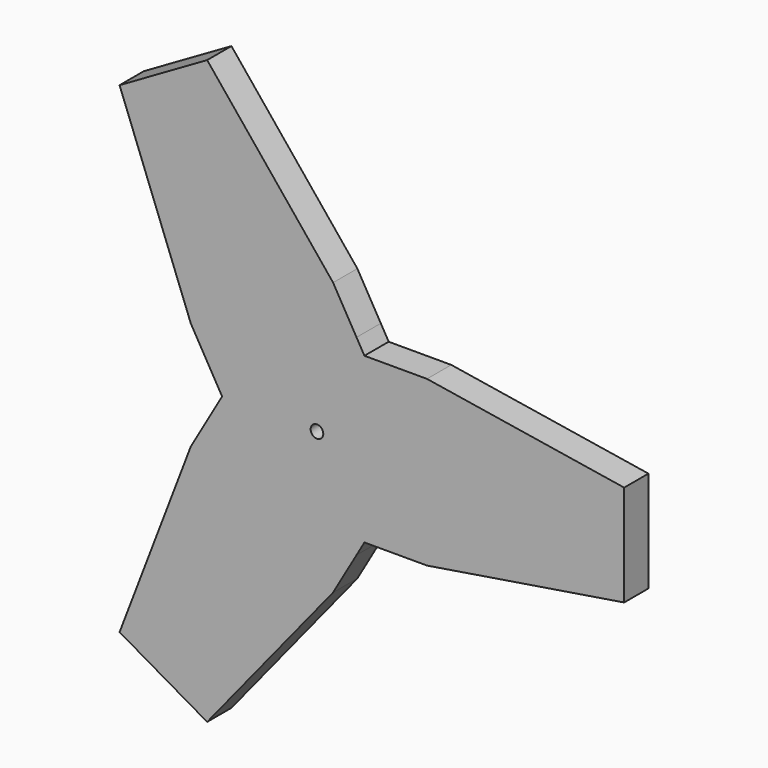
from build123d import *

# Parameters (mm, degrees)
F1_DEPTH = 6
F2_R     = 2.5
F3_DEPTH = 12.001


# Not quite as in the source:
# - a feature names something its author has since deleted; it is built from what else it names


with BuildPart() as f1:
    # F0 (on Front) → F1 (new body, symmetric)
    with BuildSketch(Plane.XZ):
        Polygon((43.524, -32.5), (121.5, -20), (121.5, 20), (43.524, 32.5), (25, 32.5), (18.7638837487, 32.5), (15.645825623, 37.9006350946), (6.383825623, 53.9428896743), (-43.4294919243, 115.2220865598), (-78.0705080757, 95.2220865598), (-49.907825623, 21.4428896743), (-40.645825623, 5.4006350946), (-37.5277674973, 0), (-40.645825623, -5.4006350946), (-49.907825623, -21.4428896743), (-78.0705080757, -95.2220865598), (-43.4294919243, -115.2220865598), (6.383825623, -53.9428896743), (15.645825623, -37.9006350946), (18.7638837487, -32.5), (25, -32.5), align=None)
    extrude(amount=F1_DEPTH, both=True)

    # F2 (on face) → F3 (cut, through all)
    with BuildSketch(Plane.XZ.offset(6)):
        Circle(F2_R)
    extrude(amount=-F3_DEPTH, mode=Mode.SUBTRACT)


solid = f1.part
